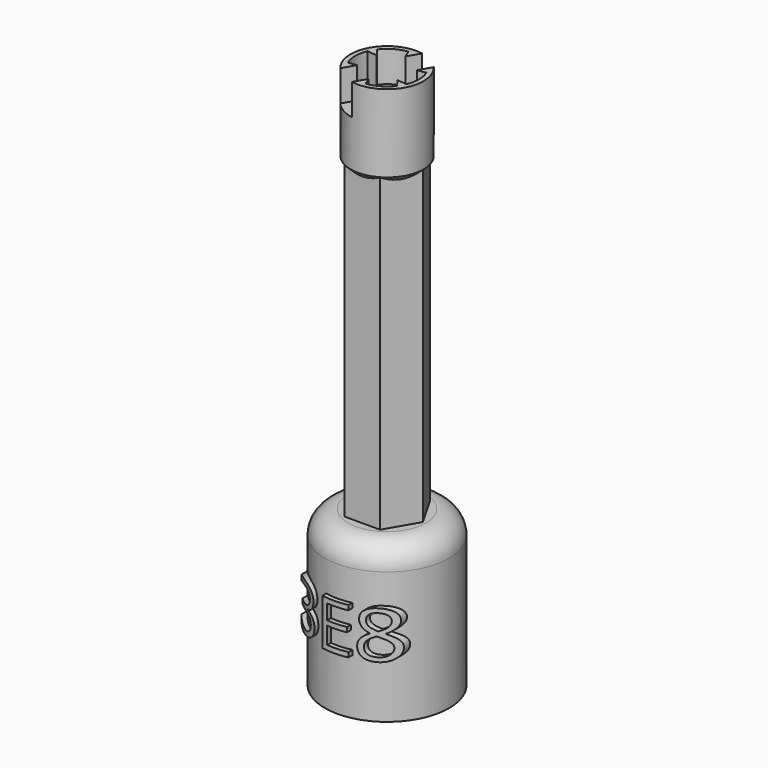
from build123d import *

# Parameters (mm, degrees)
F4_DEPTH       = 30
F5_R           = 2.35
F6_DEPTH       = 5
F8_DEPTH       = 2
F11_R          = 4
F12_DEPTH      = 10
F13_R          = 1.5
F15_W          = 1.601686293
F15_H          = 2
F16_DEPTH      = 7.3522027204
F16_DEPTH_BACK = 3.5780007331
F18_TEXT_SIZE  = 4.1666666667
F20_W          = 2.4528020591
F20_H          = 8.5


# Not quite as in the source:
# - Text() gives the source's letters only with a copy of the font that has no kerning and outlines rounded to 1/6400 em; it was checked with that copy


with BuildPart() as f4:
    # F3 (on Top) → F4 (new body)
    with BuildSketch(Plane.XY):
        Polygon((-2.3094010768, 0), (-1.1547005384, -2), (1.1547005384, -2), (2.3094010768, 0), (1.1547005384, 2), (-1.1547005384, 2), align=None)
    extrude(amount=F4_DEPTH)

    # F5 (on face) → F6 (join)
    with BuildSketch(Plane.XY.offset(30)):
        Circle(F5_R)
    extrude(amount=F6_DEPTH)

    # F7 (on face) → F8 (cut)
    with BuildSketch(Plane.XY.offset(35)):
        with BuildLine():
            ThreePointArc((1.8871010187, -0.8008431465), (2.0088625001, -0.408621409), (2.05, 0))
            ThreePointArc((2.05, 0), (2.0088625001, 0.408621409), (1.8871010187, 0.8008431465))
            Line((1.8871010187, 0.8008431465), (1.2394084499, 0.7155728022))
            Line((1.2394084499, 0.7155728022), (1.6371010187, 1.2338558484))
            ThreePointArc((1.6371010187, 1.2338558484), (1.025, 1.7753520778), (0.25, 2.0346989949))
            Line((0.25, 2.0346989949), (0, 1.4311456043))
            Line((0, 1.4311456043), (-0.25, 2.0346989949))
            ThreePointArc((-0.25, 2.0346989949), (-1.025, 1.7753520778), (-1.6371010187, 1.2338558484))
            Line((-1.6371010187, 1.2338558484), (-1.2394084499, 0.7155728022))
            Line((-1.2394084499, 0.7155728022), (-1.8871010187, 0.8008431465))
            ThreePointArc((-1.8871010187, 0.8008431465), (-2.05, 0), (-1.8871010187, -0.8008431465))
            Line((-1.8871010187, -0.8008431465), (-1.2394084499, -0.7155728022))
            Line((-1.2394084499, -0.7155728022), (-1.6371010187, -1.2338558484))
            ThreePointArc((-1.6371010187, -1.2338558484), (-1.025, -1.7753520778), (-0.25, -2.0346989949))
            Line((-0.25, -2.0346989949), (0, -1.4311456043))
            Line((0, -1.4311456043), (0.25, -2.0346989949))
            ThreePointArc((0.25, -2.0346989949), (1.025, -1.7753520778), (1.6371010187, -1.2338558484))
            Line((1.6371010187, -1.2338558484), (1.2394084499, -0.7155728022))
            Line((1.2394084499, -0.7155728022), (1.8871010187, -0.8008431465))
        make_face()
    extrude(amount=-F8_DEPTH, mode=Mode.SUBTRACT)

    # F9 (on Right) → F10 (revolve)
    with BuildSketch(Plane.YZ):
        Polygon((0, 30), (-2.35, 30), (0, 27.65), align=None)
    revolve(axis=Axis((0, 0, 15), (0, 0, -1)))

    # F11 (on face) → F12 (join)
    with BuildSketch(Plane(origin=(0, 0, 0), x_dir=(1, 0, 0), z_dir=(0, 0, -1))):
        Circle(F11_R)
    extrude(amount=-F12_DEPTH)

    # F13
    f13_edges = [f4.edges().sort_by_distance(p)[0] for p in [
        (-4, 0, 10),
    ]]
    fillet(f13_edges, radius=F13_R)

    # F15 (on 3pt) → F16 (cut, two sides)
    with BuildSketch(Plane(origin=(0.9435505093, 1.6342774217, 0), x_dir=(-0.8660254038, 0.5, 0), z_dir=(0.5, 0.8660254038, 0))) as f16_sk:
        with Locations((0, 34)):
            Rectangle(F15_W, F15_H)
    extrude(amount=-F16_DEPTH, mode=Mode.SUBTRACT)
    extrude(f16_sk.sketch, amount=F16_DEPTH_BACK, mode=Mode.SUBTRACT)

    # F18 (on offset) → F19 (join, up to the next surface of F4)
    with BuildSketch(Plane.XZ.offset(5)):
        with Locations((-3.5680338542, 3.5682411529)):
            Text('3E8', F18_TEXT_SIZE, font='Open Sans', text_align=(TextAlign.LEFT, TextAlign.BOTTOM))
    extrude(until=Until.NEXT, dir=(0, 1, 0))

    # F20 (on Front) → F21 (revolve, cut)
    with BuildSketch(Plane.XZ):
        with Locations((5.5264010295, 4.25)):
            Rectangle(F20_W, F20_H)
    revolve(axis=Axis((0, 0, 2.2814855911), (0, 0, 1)), mode=Mode.SUBTRACT)


solid = f4.part
